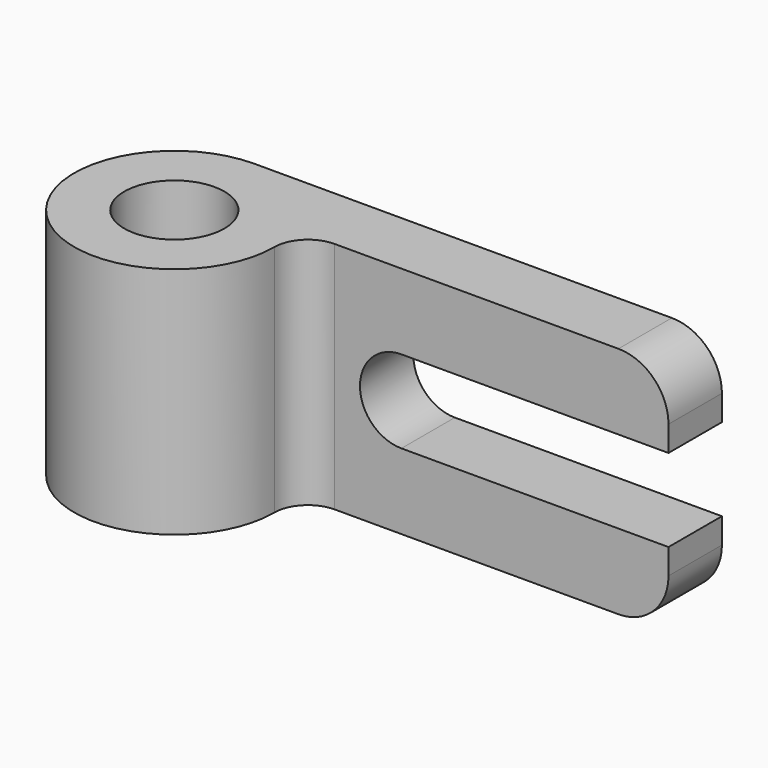
from build123d import *

# Parameters (mm, degrees)
F0_R     = 9.525
F1_DEPTH = 44.45
F3_DEPTH = 12.701
F4_R     = 6.34999
F5_R     = 9.525


# Not quite as in the source:
# - a fillet or chamfer is up to 0.001 mm smaller than in the source, because OpenCascade refuses the exact size


with BuildPart() as f1:
    # F0 (on Top) → F1 (new body)
    with BuildSketch(Plane.XY):
        with BuildLine():
            Line((88.9, 19.05), (0, 19.05))
            ThreePointArc((0, 19.05), (-13.4703841816, -13.4703841816), (19.05, 0))
            Line((19.05, 0), (19.05, 6.35))
            Line((19.05, 6.35), (88.9, 6.35))
            Line((88.9, 6.35), (88.9, 19.05))
        make_face()
        Circle(F0_R, mode=Mode.SUBTRACT)
    extrude(amount=F1_DEPTH)

    # F2 (on face) → F3 (cut, through all)
    with BuildSketch(Plane.XZ.offset(-6.35)):
        with BuildLine():
            Line((88.9, 30.099), (38.1, 30.099))
            ThreePointArc((38.1, 30.099), (30.226, 22.225), (38.1, 14.351))
            Line((38.1, 14.351), (88.9, 14.351))
            Line((88.9, 14.351), (88.9, 30.099))
        make_face()
    extrude(amount=-F3_DEPTH, mode=Mode.SUBTRACT)

    # F4 (radius 6.35 in the source; OpenCascade refuses exactly that, so slightly less here)
    f4_edges = [f1.edges().sort_by_distance(p)[0] for p in [
        (19.05, 6.35, 22.225),
    ]]
    fillet(f4_edges, radius=F4_R)

    # F5
    f5_edges = [f1.edges().sort_by_distance(p)[0] for p in [
        (88.9, 12.7, 0),
        (88.9, 12.7, 44.45),
    ]]
    fillet(f5_edges, radius=F5_R)


solid = f1.part
